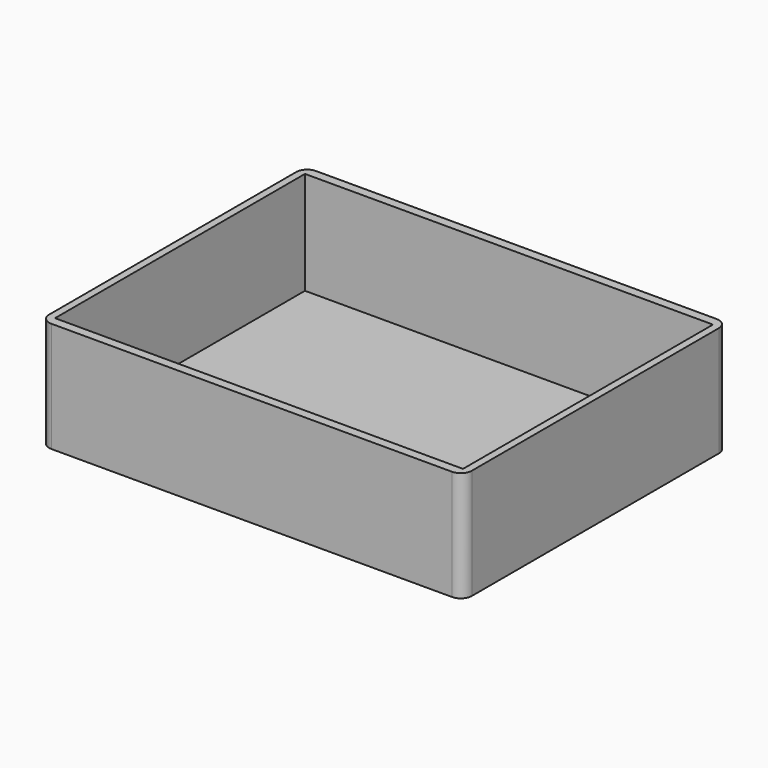
from build123d import *

# Parameters (mm, degrees)
F0_W     = 115
F0_H     = 90
F1_DEPTH = 30
F3_W     = 111
F3_H     = 85
F4_DEPTH = 28
F5_R     = 3


# Not quite as in the source:
# - a feature names something its author has since deleted; it is built from what else it names


with BuildPart() as f1:
    # F0 (on Top) → F1 (new body)
    with BuildSketch(Plane.XY):
        Rectangle(F0_W, F0_H)
    extrude(amount=F1_DEPTH)

    # F3 (on offset) → F4 (cut)
    with BuildSketch(Plane.XY.offset(30)):
        Rectangle(F3_W, F3_H)
    extrude(amount=-F4_DEPTH, mode=Mode.SUBTRACT)

    # F5
    f5_edges = [f1.edges().sort_by_distance(p)[0] for p in [
        (-57.5, 45, 15),
        (57.5, 45, 15),
        (57.5, -45, 15),
        (-57.5, -45, 15),
    ]]
    fillet(f5_edges, radius=F5_R)


solid = f1.part
